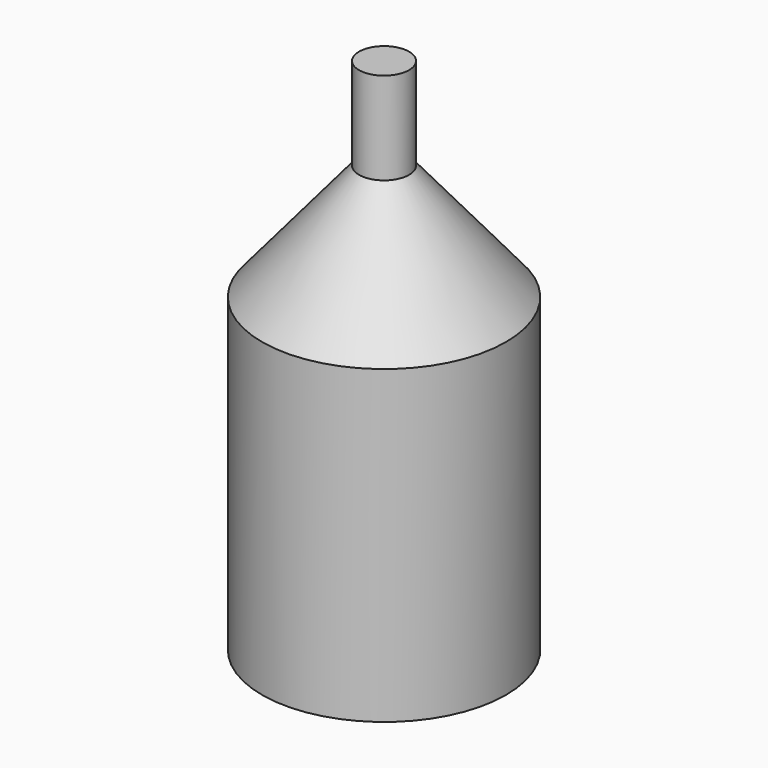
from build123d import *

# Parameters (mm, degrees)
F0_R        = 4.1
F1_DEPTH    = 15
F2_R        = 20
F3_DEPTH    = 70
F4_S5_R     = 4.1
F4_T6_DEPTH = 31


# Not quite as in the source:
# - a fillet or chamfer that OpenCascade refuses, or shapes differently, is made with other operations: its cross-section is extruded or revolved along the edge and cut away or added


with BuildPart() as f1:
    # F0 (on Top) → F1 (new body)
    with BuildSketch(Plane.XY):
        Circle(F0_R)
    extrude(amount=F1_DEPTH)

    # F2 (on Top) → F3 (join)
    with BuildSketch(Plane.XY):
        Circle(F2_R)
    extrude(amount=-F3_DEPTH)

    # F4: chamfer of 16 x 19.0680574815 on 1 edges, made by hand


with BuildPart() as f4_tool2:
    # F4_s3 → F4_t4 (revolve)
    with BuildSketch(Plane.XZ):
        Polygon((20, -19.0680574815), (4, 0), (20, 0), align=None)
    revolve(axis=Axis((0, 0, 0), (0, 0, 1)))

    # F4_s5 → F4_t6 (cut, symmetric)
    with BuildSketch(Plane.XY.offset(-9.5)):
        Circle(F4_S5_R)
    extrude(amount=F4_T6_DEPTH, both=True, mode=Mode.SUBTRACT)


with BuildPart() as f1_1:
    add(f1.part)

    # F4_t1: cut F4_tool2
    add(f4_tool2.part, mode=Mode.SUBTRACT)


solid = f1_1.part
